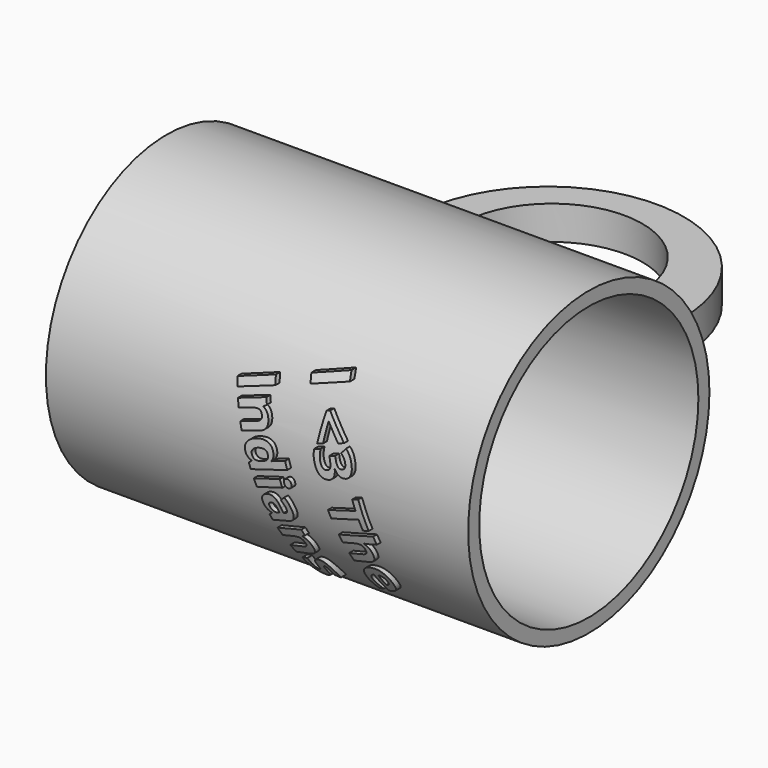
from build123d import *

# Parameters (mm, degrees)
F0_R         = 31.75
F1_DEPTH     = 88.9
F2_R         = 28.7010041845
F3_DEPTH     = 85.09
F5_DEPTH     = 7.112
F6_TEXT_SIZE = 10.7037983576
F7_DEPTH     = 34.036
F8_R         = 28.3728825393
F9_DEPTH     = 85.344
F11_DEPTH    = 64.008
F12_R        = 28.8431249381
F13_DEPTH    = 84.836


# Not quite as in the source:
# - Text() gives the source's letters only with a copy of the font that has no kerning and outlines rounded to 1/6400 em; it was checked with that copy


with BuildPart() as f1:
    # F0 (on Right) → F1 (new body)
    with BuildSketch(Plane.YZ):
        Circle(F0_R)
    extrude(amount=-F1_DEPTH)

    # F2 (on Right) → F3 (cut)
    with BuildSketch(Plane.YZ):
        Circle(F2_R)
    extrude(amount=-F3_DEPTH, mode=Mode.SUBTRACT)

    # F4 (on Top) → F5 (join)
    with BuildSketch(Plane.XY):
        with BuildLine():
            Line((-26.0949488729, 31.555917114), (-12.3693170026, 32.1080498397))
            ThreePointArc((-12.3693170026, 32.1080498397), (-40.2824425972, 67.9522197749), (-67.7314475179, 31.7514017224))
            Line((-67.7314475179, 31.7514017224), (-57.6248057187, 31.8344384432))
            ThreePointArc((-57.6248057187, 31.8344384432), (-41.596260154, 61.5378141278), (-26.0949488729, 31.555917114))
        make_face()
    extrude(amount=F5_DEPTH)

    # F6 (on Front) → F7 (join)
    with BuildSketch(Plane.XZ):
        with Locations(Location((-36.0254842499, 17.3634747101), (0, 0, -72.8162957186))):
            Text('I <3 The', F6_TEXT_SIZE, font='Open Sans', font_style=FontStyle.BOLD, text_align=(TextAlign.LEFT, TextAlign.BOTTOM))
        with Locations(Location((-49.9328534663, 13.0627588829), (0, 0, -72.8162957186))):
            Text('Indians', F6_TEXT_SIZE, font='Open Sans', font_style=FontStyle.BOLD, text_align=(TextAlign.LEFT, TextAlign.BOTTOM))
    extrude(amount=F7_DEPTH)

    # F8 (on Right) → F9 (cut)
    with BuildSketch(Plane.YZ):
        Circle(F8_R)
    extrude(amount=-F9_DEPTH, mode=Mode.SUBTRACT)

    # F10 (on Right) → F11 (cut)
    with BuildSketch(Plane.YZ):
        with BuildLine():
            ThreePointArc((29.8983208736, -13.3661104641), (-32.7395922774, -0.8255891899), (29.1866471354, 14.8560468831))
            Line((29.1866471354, 14.8560468831), (35.0276890311, 20.7231107452))
            ThreePointArc((35.0276890311, 20.7231107452), (-45.8261270879, -0.7973736558), (35.7274306521, -19.4919731381))
            Line((35.7274306521, -19.4919731381), (29.8983208736, -13.3661104641))
        make_face()
    extrude(amount=-F11_DEPTH, mode=Mode.SUBTRACT)

    # F12 (on Right) → F13 (cut)
    with BuildSketch(Plane.YZ):
        Circle(F12_R)
    extrude(amount=-F13_DEPTH, mode=Mode.SUBTRACT)


solid = f1.part
